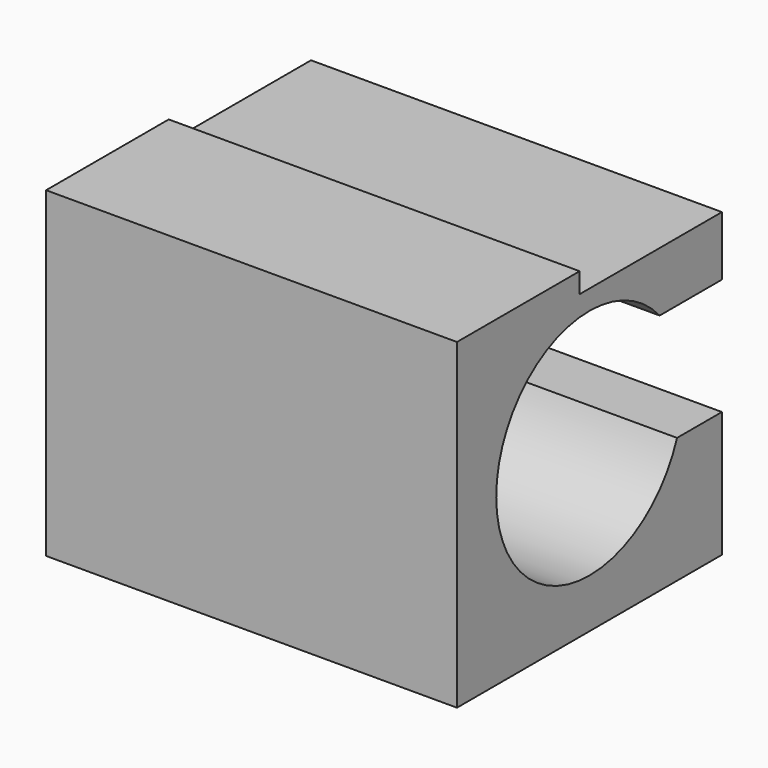
from build123d import *

# Parameters (mm, degrees)
F1_DEPTH = 67


# Not quite as in the source:
# - a feature names something its author has since deleted; it is built from what else it names


with BuildPart() as f1:
    # F0 (on Right) → F1 (new body)
    with BuildSketch(Plane.YZ):
        with BuildLine():
            Line((-23.8500006944, 31.9984000194), (-23.8500006944, -20.5015999806))
            Line((-23.8500006944, -20.5015999806), (30.1499993056, -20.5015999806))
            Line((30.1499993056, -20.5015999806), (30.1499993056, 0))
            Line((30.1499993056, 0), (21.0041528052, 0))
            ThreePointArc((21.0041528052, 0), (-15.527421475, 3.0121480227), (17.457689473, 19))
            Line((17.457689473, 19), (30.1499993056, 19))
            Line((30.1499993056, 19), (30.1499993056, 28.6984000194))
            Line((30.1499993056, 28.6984000194), (1.1499993056, 28.6984000194))
            Line((1.1499993056, 28.6984000194), (1.1499993056, 31.9984000194))
            Line((1.1499993056, 31.9984000194), (-23.8500006944, 31.9984000194))
        make_face()
    extrude(amount=F1_DEPTH)


solid = f1.part
